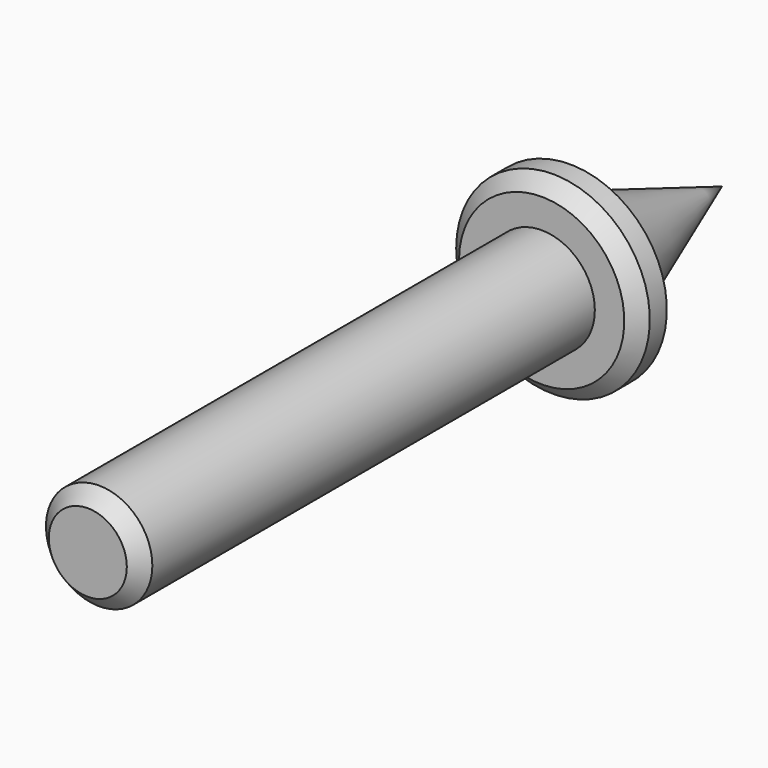
from build123d import *

# Parameters (mm, degrees)
F0_R      = 7.5
F1_DEPTH  = 80
F2_R      = 13.654
F3_DEPTH  = 5
F4_R      = 8.6540002376
F5_DEPTH  = 3
F5_FACE_R = 8.6540002376
F7_SIZE   = 2


# Not quite as in the source:
# - an extrude whose draft closes it to a point is written as a loft to that point


with BuildPart() as f1:
    # F0 (on Front) → F1 (new body)
    with BuildSketch(Plane.XZ):
        Circle(F0_R)
    extrude(amount=-F1_DEPTH)

    # F2 (on face) → F3 (join)
    with BuildSketch(Plane(origin=(0, 80, 0), x_dir=(-1, 0, 0), z_dir=(0, 1, 0))):
        Circle(F2_R)
    extrude(amount=F3_DEPTH)

    # F4 (on face) → F5 (join)
    with BuildSketch(Plane(origin=(0, 85, 0), x_dir=(-1, 0, 0), z_dir=(0, 1, 0))):
        Circle(F4_R)
    extrude(amount=F5_DEPTH)

    # F5_face (on face) → F6 section 0
    with BuildSketch(Plane(origin=(0, 88, 0), x_dir=(-1, 0, 0), z_dir=(0, 1, 0)), mode=Mode.PRIVATE) as f6_s0:
        Circle(F5_FACE_R)
    loft([f6_s0.sketch, Vertex(0, 111.7766702407, 0)], ruled=True)

    # F7
    f7_edges = [f1.edges().sort_by_distance(p)[0] for p in [
        (-7.5, 0, 0),
        (13.654, 80, 0),
    ]]
    chamfer(f7_edges, length=F7_SIZE)


solid = f1.part
